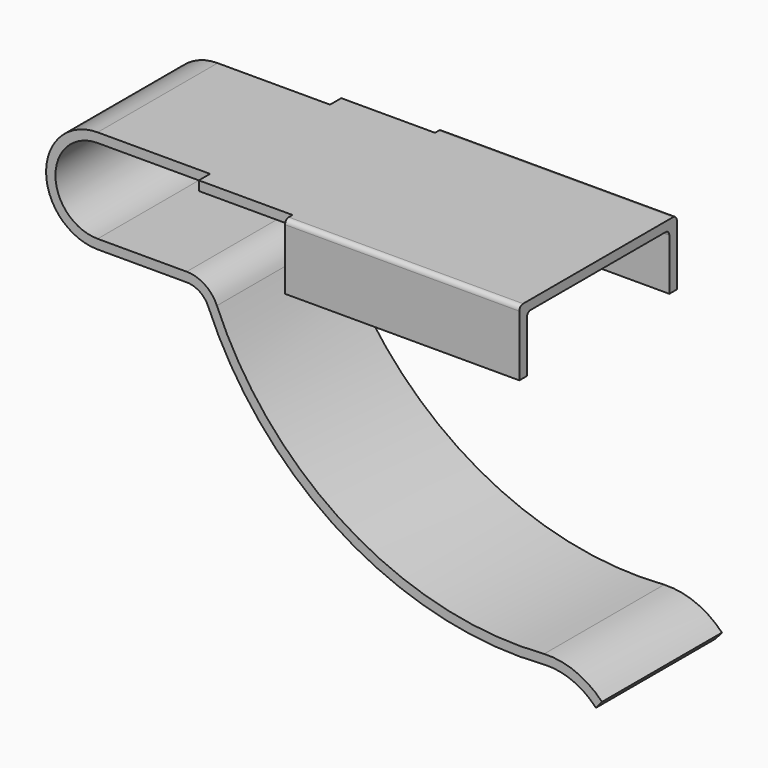
from build123d import *

# Parameters (mm, degrees)
F1_DEPTH = 16
F2_W     = 70
F2_H     = 3
F3_DEPTH = 2
F4_W     = 50
F4_H     = 14
F5_DEPTH = 2
F6_R     = 1


with BuildPart() as f1:
    # F0 (on Front) → F1 (new body)
    with BuildSketch(Plane.XZ):
        with BuildLine():
            Line((94, 11), (0, 11))
            ThreePointArc((0, 11), (-11, 0), (0, -11))
            Line((0, -11), (19, -11))
            ThreePointArc((19, -11), (21.7681124643, -11.8361612201), (23.6103896104, -14.064978646))
            ThreePointArc((23.6103896104, -14.064978646), (52.4237101957, -47.6174640031), (95.4149528414, -57.9967593826))
            ThreePointArc((95.4149528414, -57.9967593826), (101.3804745105, -59.0597282402), (106.3380534538, -62.5439444501))
            Line((106.3380534538, -62.5439444501), (107.6335766724, -61))
            ThreePointArc((107.6335766724, -61), (102.0097459375, -57.1560789275), (95.2965735981, -56))
            ThreePointArc((95.2965735981, -56), (53.4811996085, -45.9198240056), (25.4545454545, -13.2909701044))
            ThreePointArc((25.4545454545, -13.2909701044), (22.87535745, -10.1706257081), (19, -9))
            Line((19, -9), (0, -9))
            ThreePointArc((0, -9), (-9, 0), (0, 9))
            Line((0, 9), (94, 9))
            Line((94, 9), (94, 11))
        make_face()
    extrude(amount=F1_DEPTH)

    # F2 (on face) → F3 (join)
    with BuildSketch(Plane.XY.offset(11)):
        with Locations((59, -17.5)):
            Rectangle(F2_W, F2_H)
    extrude(amount=-F3_DEPTH)

    # F4 (on face) → F5 (join)
    with BuildSketch(Plane.XZ.offset(19)):
        with Locations((69, 4)):
            Rectangle(F4_W, F4_H)
    extrude(amount=F5_DEPTH)

    # F6
    f6_edges = [f1.edges().sort_by_distance(p)[0] for p in [
        (69, -21, 11),
        (69, -19, 9),
    ]]
    fillet(f6_edges, radius=F6_R)

    # F7: F1 across plane


with BuildPart() as f1_1:
    add(f1.part)
    add(f1.part.mirror(Plane.XZ))


solid = f1_1.part
